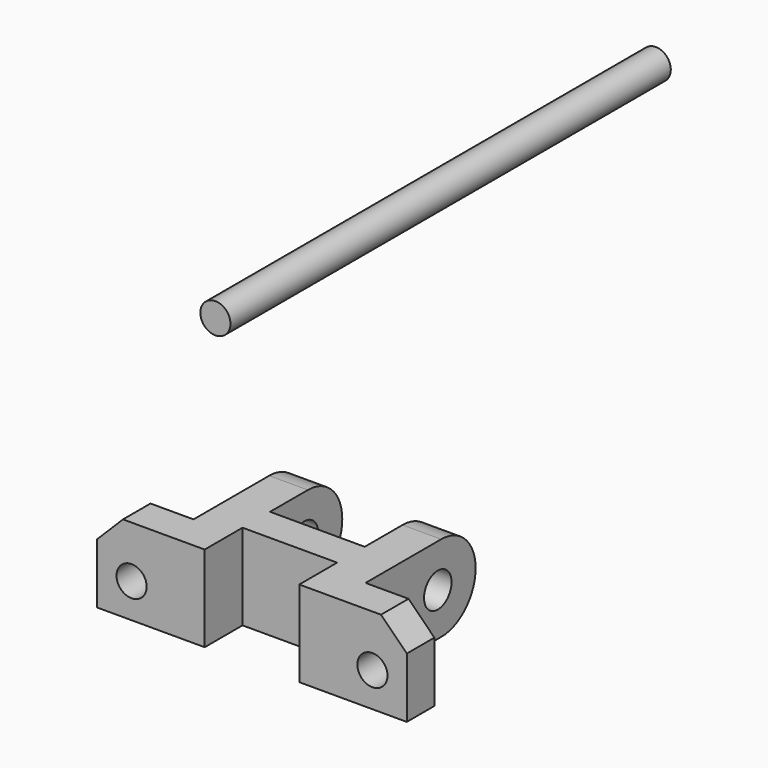
from build123d import *

# Parameters (mm, degrees)
F1_DEPTH  = 31.75
F2_R      = 6.35
F3_DEPTH  = 25.4
F4_R      = 6.35
F5_DEPTH  = 25.4
F6_R      = 5.5626
F7_DEPTH  = 25.4
F8_SIZE   = 9.525
F9_R      = 15.87499
F10_R     = 5.5626
F11_DEPTH = 203.2


# Not quite as in the source:
# - a fillet or chamfer is up to 0.001 mm smaller than in the source, because OpenCascade refuses the exact size


with BuildPart() as f1:
    # F0 (on Top) → F1 (new body)
    with BuildSketch(Plane.XY):
        Polygon((0, 17.4752), (0, 0), (39.7002, 0), (39.7002, 12.7), (14.3002, 12.7), (14.3002, 63.5), (0.0254, 63.5), (0.0254, 30.1752), (-34.925, 30.1752), (-34.925, 63.5), (-49.1998, 63.5), (-49.1998, 12.7), (-74.5998, 12.7), (-74.5998, 0), (-34.925, 0), (-34.925, 17.4752), align=None)
    extrude(amount=-F1_DEPTH)

    # F2 (on face) → F3 (cut)
    with BuildSketch(Plane.YZ.offset(14.3002)):
        with Locations((46.0502, -15.875)):
            Circle(F2_R)
    extrude(amount=-F3_DEPTH, mode=Mode.SUBTRACT)

    # F4 (on face) → F5 (cut)
    with BuildSketch(Plane(origin=(-49.1998, 0, 0), x_dir=(0, -1, 0), z_dir=(-1, 0, 0))):
        with Locations((-46.0502, -15.875)):
            Circle(F4_R)
    extrude(amount=-F5_DEPTH, mode=Mode.SUBTRACT)

    # F6 (on face) → F7 (cut)
    with BuildSketch(Plane(origin=(0, 12.7, 0), x_dir=(-1, 0, 0), z_dir=(0, 1, 0))):
        with Locations((61.8998, -19.05)):
            Circle(F6_R)
        with Locations((-27.0002, -19.05)):
            Circle(F6_R)
    extrude(amount=-F7_DEPTH, mode=Mode.SUBTRACT)

    # F8
    f8_edges = [f1.edges().sort_by_distance(p)[0] for p in [
        (-74.5998, 6.35, 0),
        (39.7002, 6.35, 0),
    ]]
    chamfer(f8_edges, length=F8_SIZE)

    # F9 (radius 15.875 in the source; OpenCascade refuses exactly that, so slightly less here)
    f9_edges = [f1.edges().sort_by_distance(p)[0] for p in [
        (-42.0624, 63.5, 0),
        (-42.0624, 63.5, -31.75),
        (7.1628, 63.5, -31.75),
        (7.1628, 63.5, 0),
    ]]
    fillet(f9_edges, radius=F9_R)


with BuildPart() as f11:
    # F10 (on Front) → F11 (new body)
    with BuildSketch(Plane.XZ):
        with Locations((-30.9646371752, 76.4614716172)):
            Circle(F10_R)
    extrude(amount=-F11_DEPTH)


solid = Compound([f1.part, f11.part])
